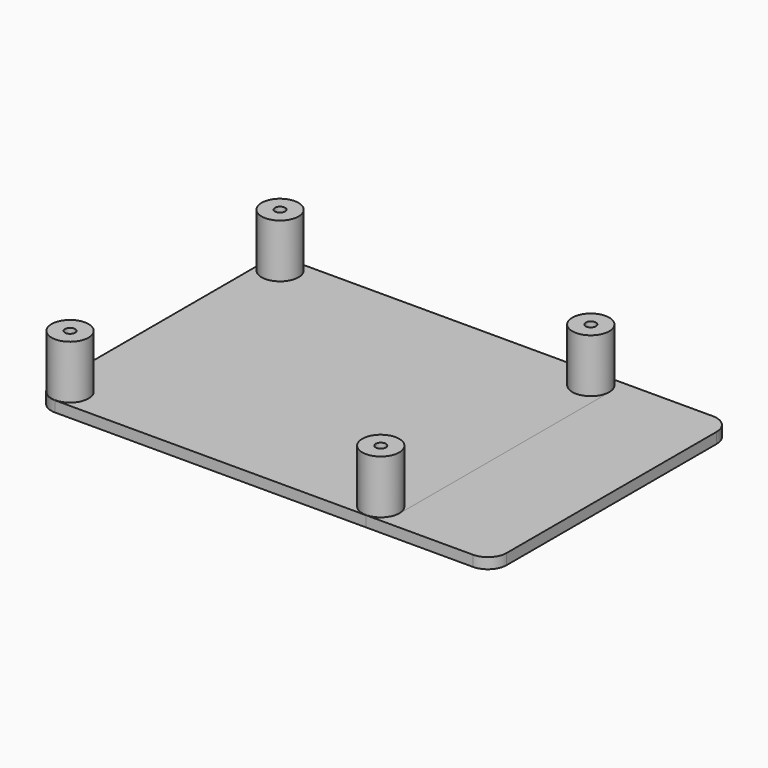
from build123d import *

# Parameters (mm, degrees)
F0_R     = 3.45
F0_R_2   = 2.25
F2_DEPTH = 2
F0_R_3   = 0.95
F3_DEPTH = 7
F1_R     = 3.45
F1_R_2   = 2.25
F4_DEPTH = 2
F1_R_3   = 0.95
F5_DEPTH = 12
F6_DEPTH = 4
F7_DEPTH = 5


with BuildPart() as f2:
    # F0 (on Top) → F2 (new body)
    with BuildSketch(Plane.XY):
        with BuildLine():
            ThreePointArc((0, 3.5), (1.0251262658, 1.0251262658), (3.5, 0))
            Line((3.5, 0), (81.5, 0))
            ThreePointArc((81.5, 0), (83.9748737342, 1.0251262658), (85, 3.5))
            Line((85, 3.5), (85, 52.5))
            ThreePointArc((85, 52.5), (83.9748737342, 54.9748737342), (81.5, 56))
            Line((81.5, 56), (3.5, 56))
            ThreePointArc((3.5, 56), (1.0251262658, 54.9748737342), (0, 52.5))
            Line((0, 52.5), (0, 3.5))
        make_face()
        with Locations((3.5, 3.5)):
            Circle(F0_R, mode=Mode.SUBTRACT)
        with Locations((61.5, 3.5)):
            Circle(F0_R, mode=Mode.SUBTRACT)
        with Locations((3.5, 52.5)):
            Circle(F0_R, mode=Mode.SUBTRACT)
        with Locations((61.5, 52.5)):
            Circle(F0_R, mode=Mode.SUBTRACT)
        with Locations((3.5, 52.5)):
            Circle(F0_R)
        with Locations((3.5, 52.5)):
            Circle(F0_R_2, mode=Mode.SUBTRACT)
        with Locations((61.5, 52.5)):
            Circle(F0_R)
        with Locations((61.5, 52.5)):
            Circle(F0_R_2, mode=Mode.SUBTRACT)
        with Locations((61.5, 3.5)):
            Circle(F0_R)
        with Locations((61.5, 3.5)):
            Circle(F0_R_2, mode=Mode.SUBTRACT)
        with Locations((3.5, 3.5)):
            Circle(F0_R)
        with Locations((3.5, 3.5)):
            Circle(F0_R_2, mode=Mode.SUBTRACT)
    extrude(amount=F2_DEPTH)

    # F0 (on Top) → F3 (join)
    with BuildSketch(Plane.XY):
        with Locations((3.5, 3.5)):
            Circle(F0_R)
        with Locations((3.5, 3.5)):
            Circle(F0_R_2, mode=Mode.SUBTRACT)
        with Locations((3.5, 52.5)):
            Circle(F0_R)
        with Locations((3.5, 52.5)):
            Circle(F0_R_2, mode=Mode.SUBTRACT)
        with Locations((61.5, 3.5)):
            Circle(F0_R)
        with Locations((61.5, 3.5)):
            Circle(F0_R_2, mode=Mode.SUBTRACT)
        with Locations((61.5, 52.5)):
            Circle(F0_R)
        with Locations((61.5, 52.5)):
            Circle(F0_R_2, mode=Mode.SUBTRACT)
        with Locations((61.5, 52.5)):
            Circle(F0_R_2)
        with Locations((61.5, 52.5)):
            Circle(F0_R_3, mode=Mode.SUBTRACT)
        with Locations((61.5, 3.5)):
            Circle(F0_R_2)
        with Locations((61.5, 3.5)):
            Circle(F0_R_3, mode=Mode.SUBTRACT)
        with Locations((3.5, 3.5)):
            Circle(F0_R_2)
        with Locations((3.5, 3.5)):
            Circle(F0_R_3, mode=Mode.SUBTRACT)
        with Locations((3.5, 52.5)):
            Circle(F0_R_2)
        with Locations((3.5, 52.5)):
            Circle(F0_R_3, mode=Mode.SUBTRACT)
    extrude(amount=F3_DEPTH)


with BuildPart() as f4:
    # F1 (on Top) → F4 (new body)
    with BuildSketch(Plane.XY):
        with BuildLine():
            ThreePointArc((0, 3.5), (1.0251262658, 1.0251262658), (3.5, 0))
            Line((3.5, 0), (61.5, 0))
            ThreePointArc((61.5, 0), (63.9748737342, 1.0251262658), (65, 3.5))
            Line((65, 3.5), (65, 52.5))
            ThreePointArc((65, 52.5), (63.9748737342, 54.9748737342), (61.5, 56))
            Line((61.5, 56), (3.5, 56))
            ThreePointArc((3.5, 56), (1.0251262658, 54.9748737342), (0, 52.5))
            Line((0, 52.5), (0, 3.5))
        make_face()
        with Locations((3.5, 3.5)):
            Circle(F1_R, mode=Mode.SUBTRACT)
        with Locations((61.5, 3.5)):
            Circle(F1_R, mode=Mode.SUBTRACT)
        with Locations((3.5, 52.5)):
            Circle(F1_R, mode=Mode.SUBTRACT)
        with Locations((61.5, 52.5)):
            Circle(F1_R, mode=Mode.SUBTRACT)
        with Locations((3.5, 3.5)):
            Circle(F1_R)
        with Locations((3.5, 3.5)):
            Circle(F1_R_2, mode=Mode.SUBTRACT)
        with Locations((61.5, 3.5)):
            Circle(F1_R)
        with Locations((61.5, 3.5)):
            Circle(F1_R_2, mode=Mode.SUBTRACT)
        with Locations((3.5, 52.5)):
            Circle(F1_R)
        with Locations((3.5, 52.5)):
            Circle(F1_R_2, mode=Mode.SUBTRACT)
        with Locations((61.5, 52.5)):
            Circle(F1_R)
        with Locations((61.5, 52.5)):
            Circle(F1_R_2, mode=Mode.SUBTRACT)
    extrude(amount=F4_DEPTH)

    # F1 (on Top) → F5 (join)
    with BuildSketch(Plane.XY):
        with Locations((61.5, 3.5)):
            Circle(F1_R)
        with Locations((61.5, 3.5)):
            Circle(F1_R_2, mode=Mode.SUBTRACT)
        with Locations((3.5, 3.5)):
            Circle(F1_R)
        with Locations((3.5, 3.5)):
            Circle(F1_R_2, mode=Mode.SUBTRACT)
        with Locations((3.5, 52.5)):
            Circle(F1_R)
        with Locations((3.5, 52.5)):
            Circle(F1_R_2, mode=Mode.SUBTRACT)
        with Locations((61.5, 52.5)):
            Circle(F1_R)
        with Locations((61.5, 52.5)):
            Circle(F1_R_2, mode=Mode.SUBTRACT)
        with Locations((61.5, 3.5)):
            Circle(F1_R_2)
        with Locations((61.5, 3.5)):
            Circle(F1_R_3, mode=Mode.SUBTRACT)
        with Locations((3.5, 3.5)):
            Circle(F1_R_2)
        with Locations((3.5, 3.5)):
            Circle(F1_R_3, mode=Mode.SUBTRACT)
        with Locations((3.5, 52.5)):
            Circle(F1_R_2)
        with Locations((3.5, 52.5)):
            Circle(F1_R_3, mode=Mode.SUBTRACT)
        with Locations((61.5, 52.5)):
            Circle(F1_R_2)
        with Locations((61.5, 52.5)):
            Circle(F1_R_3, mode=Mode.SUBTRACT)
    extrude(amount=F5_DEPTH)


with BuildPart() as f6_tool:
    # F0 (on Top) → F6 (new body)
    with BuildSketch(Plane.XY):
        with Locations((61.5, 3.5)):
            Circle(F0_R_2)
        with Locations((61.5, 3.5)):
            Circle(F0_R_3, mode=Mode.SUBTRACT)
        with Locations((61.5, 52.5)):
            Circle(F0_R_2)
        with Locations((61.5, 52.5)):
            Circle(F0_R_3, mode=Mode.SUBTRACT)
        with Locations((3.5, 52.5)):
            Circle(F0_R_2)
        with Locations((3.5, 52.5)):
            Circle(F0_R_3, mode=Mode.SUBTRACT)
        with Locations((3.5, 3.5)):
            Circle(F0_R_2)
        with Locations((3.5, 3.5)):
            Circle(F0_R_3, mode=Mode.SUBTRACT)
        with Locations((61.5, 3.5)):
            Circle(F0_R_3)
        with Locations((61.5, 52.5)):
            Circle(F0_R_3)
        with Locations((3.5, 52.5)):
            Circle(F0_R_3)
        with Locations((3.5, 3.5)):
            Circle(F0_R_3)
    extrude(amount=F6_DEPTH)


with BuildPart() as f2_1:
    add(f2.part)

    # F6: cut by f6_tool
    add(f6_tool.part, mode=Mode.SUBTRACT)


with BuildPart() as f4_1:
    add(f4.part)

    # F6: cut by f6_tool
    add(f6_tool.part, mode=Mode.SUBTRACT)

    # F1 (on Top) → F7 (cut)
    with BuildSketch(Plane.XY):
        with Locations((61.5, 3.5)):
            Circle(F1_R_2)
        with Locations((61.5, 3.5)):
            Circle(F1_R_3, mode=Mode.SUBTRACT)
        with Locations((61.5, 3.5)):
            Circle(F1_R_3)
        with Locations((3.5, 3.5)):
            Circle(F1_R_2)
        with Locations((3.5, 3.5)):
            Circle(F1_R_3, mode=Mode.SUBTRACT)
        with Locations((3.5, 3.5)):
            Circle(F1_R_3)
        with Locations((3.5, 52.5)):
            Circle(F1_R_2)
        with Locations((3.5, 52.5)):
            Circle(F1_R_3, mode=Mode.SUBTRACT)
        with Locations((3.5, 52.5)):
            Circle(F1_R_3)
        with Locations((61.5, 52.5)):
            Circle(F1_R_2)
        with Locations((61.5, 52.5)):
            Circle(F1_R_3, mode=Mode.SUBTRACT)
        with Locations((61.5, 52.5)):
            Circle(F1_R_3)
    extrude(amount=F7_DEPTH, mode=Mode.SUBTRACT)


solid = Compound([f2_1.part, f4_1.part])
